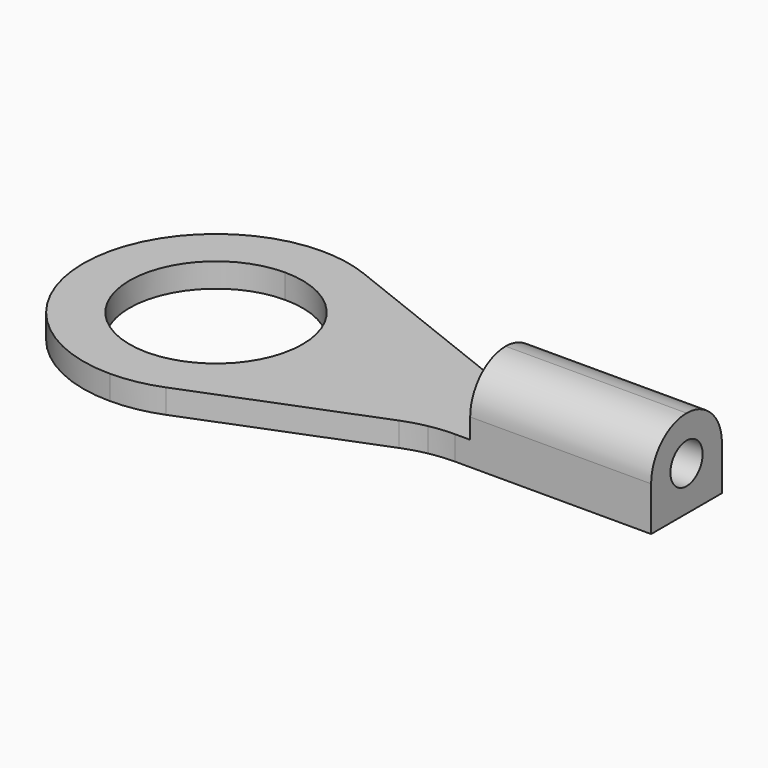
from build123d import *

# Parameters (mm, degrees)
F0_W     = 4.5
F0_H     = 2.2
F1_DEPTH = 0.6
F2_W     = 4.5
F2_H     = 2.2
F3_DEPTH = 1.6
F4_R     = 1.09999
F5_R     = 0.5
F6_DEPTH = 25


# Not quite as in the source:
# - a fillet or chamfer is up to 0.001 mm smaller than in the source, because OpenCascade refuses the exact size


with BuildPart() as f1:
    # F0 (on Top) → F1 (new body)
    with BuildSketch(Plane.XY):
        with BuildLine():
            ThreePointArc((8.9159970588, 1.9694225865), (9.2040660975, 2.0680561106), (9.5, 2.1397182935))
            Line((9.5, 2.1397182935), (9.5, 4.4602817065))
            ThreePointArc((9.5, 4.4602817065), (9.2040660975, 4.5319438894), (8.9159970588, 4.6305774135))
            Line((8.9159970588, 4.6305774135), (4.5118766379, 6.3694225865))
            ThreePointArc((4.5118766379, 6.3694225865), (3.9168085053, 6.5418431899), (3.3, 6.6))
            Line((3.3, 6.6), (3.3, 5.45))
            ThreePointArc((3.3, 5.45), (4.8202795796, 4.8202795796), (5.45, 3.3))
            ThreePointArc((5.45, 3.3), (4.8202795796, 1.7797204204), (3.3, 1.15))
            Line((3.3, 1.15), (3.3, 0))
            ThreePointArc((3.3, 0), (3.9168085053, 0.0581568101), (4.5118766379, 0.2305774135))
            Line((4.5118766379, 0.2305774135), (8.9159970588, 1.9694225865))
        make_face()
        with Locations((12.75, 3.3)):
            Rectangle(F0_W, F0_H)
        with BuildLine():
            Line((10.1278736967, 2.2), (10.5, 2.2))
            Line((10.5, 2.2), (10.5, 4.4))
            Line((10.5, 4.4), (10.1278736967, 4.4))
            ThreePointArc((10.1278736967, 4.4), (9.8124932664, 4.4151049965), (9.5, 4.4602817065))
            Line((9.5, 4.4602817065), (9.5, 2.1397182935))
            ThreePointArc((9.5, 2.1397182935), (9.8124932664, 2.1848950035), (10.1278736967, 2.2))
        make_face()
        with BuildLine():
            ThreePointArc((0, 3.3), (0.9665476221, 0.9665476221), (3.3, 0))
            Line((3.3, 0), (3.3, 1.15))
            ThreePointArc((3.3, 1.15), (1.15, 3.3), (3.3, 5.45))
            Line((3.3, 5.45), (3.3, 6.6))
            ThreePointArc((3.3, 6.6), (0.9665476221, 5.6334523779), (0, 3.3))
        make_face()
    extrude(amount=F1_DEPTH)

    # F2 (on face) → F3 (join)
    with BuildSketch(Plane.XY.offset(0.6)):
        with Locations((12.75, 3.3)):
            Rectangle(F2_W, F2_H)
    extrude(amount=F3_DEPTH)

    # F4 (radius 1.1 in the source; OpenCascade refuses exactly that, so slightly less here)
    f4_edges = [f1.edges().sort_by_distance(p)[0] for p in [
        (12.75, 4.4, 2.2),
        (12.75, 2.2, 2.2),
    ]]
    fillet(f4_edges, radius=F4_R)

    # F5 (on face) → F6 (cut)
    with BuildSketch(Plane.YZ.offset(15)):
        with Locations((3.3, 1.1)):
            Circle(F5_R)
    extrude(amount=-F6_DEPTH, mode=Mode.SUBTRACT)


solid = f1.part
